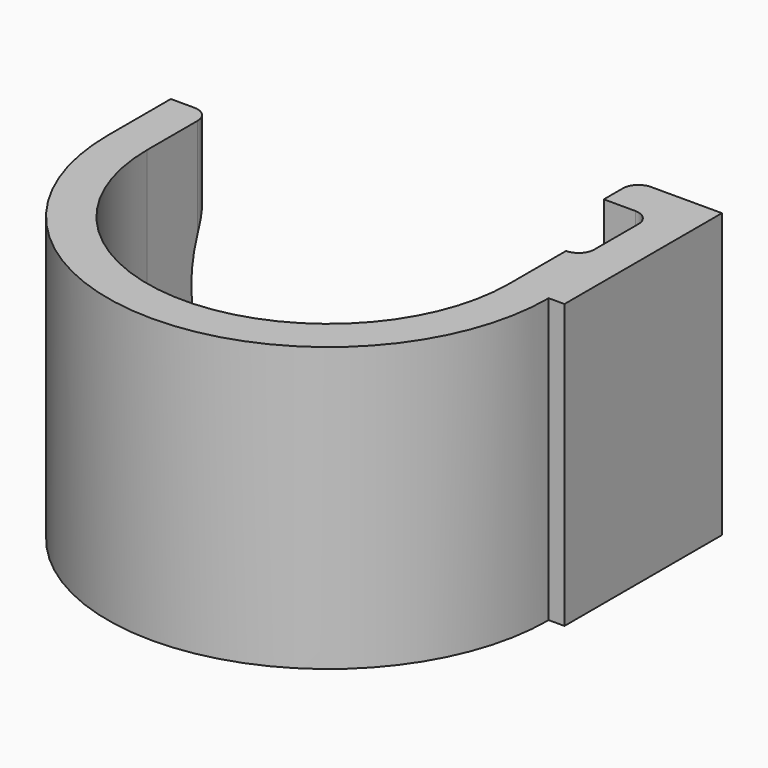
from build123d import *

# Parameters (mm, degrees)
F1_DEPTH = 18
F2_R     = 7.5
F3_DEPTH = 19.001
F4_R     = 7.5
F5_DEPTH = 25
F6_R     = 0.99999


# Not quite as in the source:
# - a fillet or chamfer is up to 0.001 mm smaller than in the source, because OpenCascade refuses the exact size


with BuildPart() as f1:
    # F0 (on Top) → F1 (new body)
    with BuildSketch(Plane.XY):
        with BuildLine():
            ThreePointArc((11.5, 0), (0, -11.5), (-11.5, 0))
            Line((-11.5, 0), (-11.5, 5))
            Line((-11.5, 5), (-14, 5))
            Line((-14, 5), (-14, 0))
            ThreePointArc((-14, 0), (0, -14), (14, 0))
            Line((14, 0), (15, 0))
            Line((15, 0), (15, 12.5))
            Line((15, 12.5), (9.5, 12.5))
            Line((9.5, 12.5), (9.5, 10))
            Line((9.5, 10), (12.5, 10))
            Line((12.5, 10), (12.5, 4.5))
            Line((12.5, 4.5), (11.5, 4.5))
            Line((11.5, 4.5), (11.5, 0))
        make_face()
    extrude(amount=F1_DEPTH)

    # F2 (on face) → F3 (cut, through all)
    with BuildSketch(Plane(origin=(0, 5, 0), x_dir=(-1, 0, 0), z_dir=(0, 1, 0))):
        with Locations((20, 9)):
            Circle(F2_R)
    extrude(amount=-F3_DEPTH, mode=Mode.SUBTRACT)

    # F4 (on face) → F5 (cut)
    with BuildSketch(Plane.YZ.offset(-11.5)):
        with Locations((11, 9)):
            Circle(F4_R)
    extrude(amount=-F5_DEPTH, mode=Mode.SUBTRACT)

    # F6 (radius 1 in the source; OpenCascade refuses exactly that, so slightly less here)
    f6_edges = [f1.edges().sort_by_distance(p)[0] for p in [
        (-11.5, 5, 15.75),
        (-11.5, 5, 2.25),
        (12.5, 4.5, 9),
        (12.5, 10, 9),
        (9.5, 12.5, 9),
    ]]
    fillet(f6_edges, radius=F6_R)


solid = f1.part
